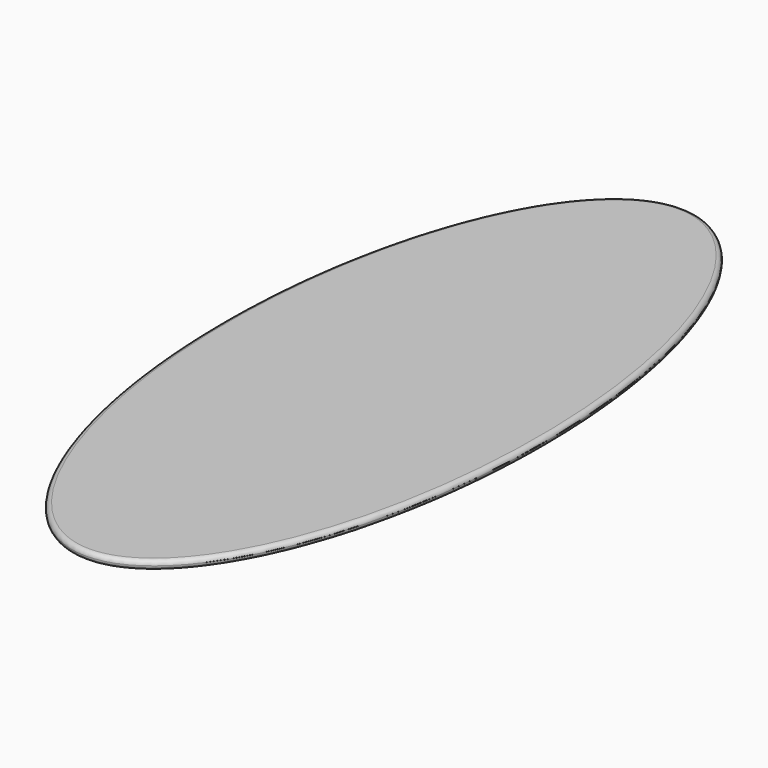
from build123d import *

# Parameters (mm, degrees)
F1_DEPTH  = 31.75
F3_DEPTH  = 19.05
F4_R      = 19.04999
F5_R      = 6.34999
F6_R      = 8.73125
F7_R      = 8.73125
F9_R      = 8.73125
F8_R      = 8.73125
F10_DEPTH = 19.05


# Not quite as in the source:
# - a fillet or chamfer is up to 0.001 mm smaller than in the source, because OpenCascade refuses the exact size


with BuildPart() as f1:
    # F0 (on Top) → F1 (new body)
    with BuildSketch(Plane.XY):
        with BuildLine():
            add(Edge.make_bspline(
                [(0, -533.4), (395.9468146102, -533.4), (197.9734073051, 266.7), (0, 1066.8), (-197.9734073051, 266.7), (-395.9468146102, -533.4), (0, -533.4)],
                knots=[0, 0, 0, 2.0943951024, 2.0943951024, 4.1887902048, 4.1887902048, 6.2831853072, 6.2831853072, 6.2831853072], degree=2, weights=[1, 0.5, 1, 0.5, 1, 0.5, 1]))
        make_face()
    extrude(amount=F1_DEPTH)

    # F2 (on face) → F3 (cut)
    with BuildSketch(Plane(origin=(0, 0, 0), x_dir=(1, 0, 0), z_dir=(0, 0, -1))):
        with BuildLine():
            add(Edge.make_bspline(
                [(0, 533.4), (395.9468146102, 533.4), (197.9734073051, -266.7), (0, -1066.8), (-197.9734073051, -266.7), (-395.9468146102, 533.4), (0, 533.4)],
                knots=[0, 0, 0, 2.0943951024, 2.0943951024, 4.1887902048, 4.1887902048, 6.2831853072, 6.2831853072, 6.2831853072], degree=2, weights=[1, 0.5, 1, 0.5, 1, 0.5, 1]))
        make_face()
        with BuildLine():
            ThreePointArc((-127, 252.4125), (-146.0830442573, 298.4830442573), (-100.0125, 279.4))
            Line((-100.0125, 279.4), (100.0125, 279.4))
            ThreePointArc((100.0125, 279.4), (127, 306.3875), (153.9875, 279.4))
            ThreePointArc((153.9875, 279.4), (146.0830442573, 260.3169557427), (127, 252.4125))
            Line((127, 252.4125), (127, -252.4125))
            ThreePointArc((127, -252.4125), (146.0830442573, -260.3169557427), (153.9875, -279.4))
            ThreePointArc((153.9875, -279.4), (127, -306.3875), (100.0125, -279.4))
            Line((100.0125, -279.4), (-100.0125, -279.4))
            ThreePointArc((-100.0125, -279.4), (-146.0830442573, -298.4830442573), (-127, -252.4125))
            Line((-127, -252.4125), (-127, 252.4125))
        make_face(mode=Mode.SUBTRACT)
        with BuildLine():
            Line((100.0125, 279.4), (-100.0125, 279.4))
            ThreePointArc((-100.0125, 279.4), (-107.9169557427, 260.3169557427), (-127, 252.4125))
            Line((-127, 252.4125), (-127, -252.4125))
            ThreePointArc((-127, -252.4125), (-107.9169557427, -260.3169557427), (-100.0125, -279.4))
            Line((-100.0125, -279.4), (100.0125, -279.4))
            ThreePointArc((100.0125, -279.4), (107.9169557427, -260.3169557427), (127, -252.4125))
            Line((127, -252.4125), (127, 252.4125))
            ThreePointArc((127, 252.4125), (107.9169557427, 260.3169557427), (100.0125, 279.4))
        make_face()
    extrude(amount=-F3_DEPTH, mode=Mode.SUBTRACT)

    # F4 (radius 19.05 in the source; OpenCascade refuses exactly that, so slightly less here)
    f4_edges = [f1.edges().sort_by_distance(p)[0] for p in [
        (127, -306.3875, 19.05),
        (-153.9875, -279.4, 19.05),
        (153.9875, 279.4, 19.05),
        (-127, 306.3875, 19.05),
    ]]
    fillet(f4_edges, radius=F4_R)

    # F5 (radius 6.35 in the source; OpenCascade refuses exactly that, so slightly less here)
    f5_edges = [f1.edges().sort_by_distance(p)[0] for p in [
        (0.000353, 533.4, 31.75),
        (0.000353, 533.4, 19.05),
    ]]
    fillet(f5_edges, radius=F5_R)

    # F6 (on face) + F7 (on face) + F9 (on face) + F8 (on face) → F10 (cut)
    with BuildSketch(Plane(origin=(0, 0, 0), x_dir=(1, 0, 0), z_dir=(0, 0, -1))):
        with Locations((-127, -279.4)):
            Circle(F6_R)
    with BuildSketch(Plane(origin=(0, 0, 0), x_dir=(1, 0, 0), z_dir=(0, 0, -1))):
        with Locations((-127, 279.4)):
            Circle(F7_R)
    with BuildSketch(Plane(origin=(0, 0, 0), x_dir=(1, 0, 0), z_dir=(0, 0, -1))):
        with Locations((127, 279.4)):
            Circle(F9_R)
    with BuildSketch(Plane(origin=(0, 0, 0), x_dir=(1, 0, 0), z_dir=(0, 0, -1))):
        with Locations((127, -279.4)):
            Circle(F8_R)
    extrude(amount=-F10_DEPTH, mode=Mode.SUBTRACT)


solid = f1.part
